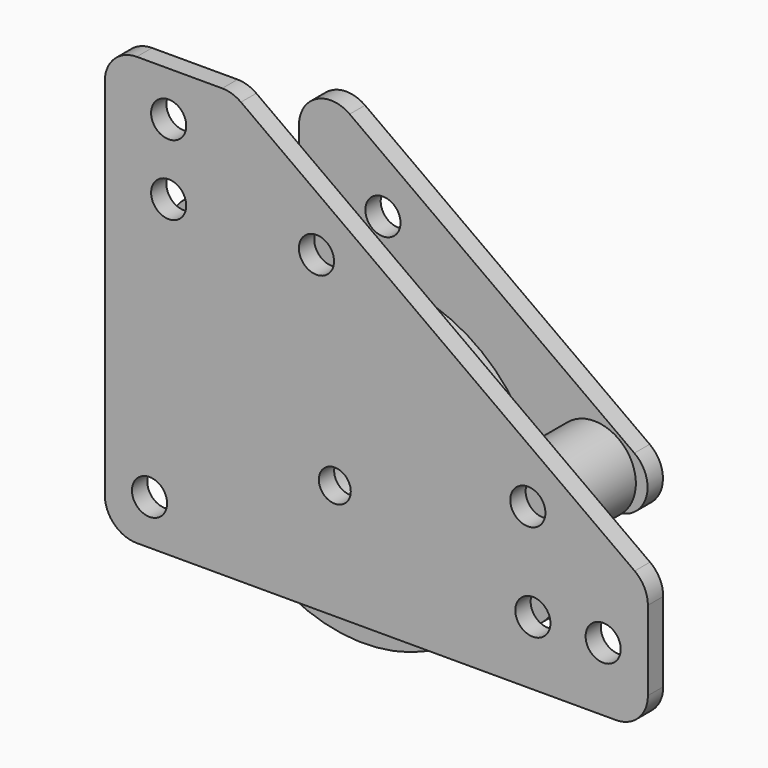
from build123d import *

# Parameters (mm, degrees)
F0_R      = 20
F0_R_2    = 13
F1_DEPTH  = 5
F0_R_3    = 24
F2_DEPTH  = 2.4
F4_R      = 2.75
F4_R_2    = 2.5
F5_DEPTH  = 3
F6_R      = 13
F6_R_2    = 5
F7_DEPTH  = 8
F8_R      = 2.75
F9_DEPTH  = 3
F10_R     = 5
F10_2_R   = 5
F11_R     = 6.5
F12_DEPTH = 10


# Not quite as in the source:
# - a feature names something its author has since deleted; it is built from what else it names


with BuildPart() as f1:
    # F0 (on Front) → F1 (new body, symmetric)
    with BuildSketch(Plane.XZ):
        Circle(F0_R)
        Circle(F0_R_2, mode=Mode.SUBTRACT)
    extrude(amount=F1_DEPTH, both=True)

    # F0 (on Front) → F2 (join, symmetric)
    with BuildSketch(Plane.XZ):
        Circle(F0_R_3)
        Circle(F0_R, mode=Mode.SUBTRACT)
    extrude(amount=F2_DEPTH, both=True)


with BuildPart() as f5:
    # F4 (on offset) → F5 (new body)
    with BuildSketch(Plane.XZ.offset(5)):
        Polygon((-16, 49), (-36, 49), (-36, -18), (49, -18), (49, 2), align=None)
        with Locations((-28.9929573972, -10.9929573972)):
            Circle(F4_R, mode=Mode.SUBTRACT)
        Circle(F4_R_2, mode=Mode.SUBTRACT)
        with Locations((31, -8)):
            Circle(F4_R, mode=Mode.SUBTRACT)
        with Locations((42, -8)):
            Circle(F4_R, mode=Mode.SUBTRACT)
        with Locations((30.2115080133, 6.9472860574)):
            Circle(F4_R, mode=Mode.SUBTRACT)
        with Locations((-26, 31)):
            Circle(F4_R, mode=Mode.SUBTRACT)
        with Locations((-2.8688968517, 30.8669634213)):
            Circle(F4_R, mode=Mode.SUBTRACT)
        with Locations((-26, 42)):
            Circle(F4_R, mode=Mode.SUBTRACT)
    extrude(amount=F5_DEPTH)

    # F10#2
    f10_2_edges = [f5.edges().sort_by_distance(p)[0] for p in [
        (-36, -6.5, 49),
        (-36, -6.5, -18),
        (49, -6.5, -18),
        (49, -6.5, 2),
        (-16, -6.5, 49),
    ]]
    fillet(f10_2_edges, radius=F10_2_R)


with BuildPart() as f7:
    # F6 (on offset) → F7 (new body)
    with BuildSketch(Plane.XZ.offset(5)):
        Circle(F6_R)
        Circle(F6_R_2, mode=Mode.SUBTRACT)
    extrude(amount=-F7_DEPTH)


with BuildPart() as f9:
    # F8 (on face) → F9 (new body)
    with BuildSketch(Plane(origin=(0, 5, 0), x_dir=(-1, 0, 0), z_dir=(0, 1, 0))):
        Polygon((-24, 2), (-24, -18), (36, -18), (36, 24), (16, 24), (16, 49), (-49, 2), align=None)
        with Locations((-30.2115080133, 6.9472860574)):
            Circle(F8_R, mode=Mode.SUBTRACT)
        with Locations((28.9929573972, -10.9929573972)):
            Circle(F8_R, mode=Mode.SUBTRACT)
        with Locations((2.8688968517, 30.8669634213)):
            Circle(F8_R, mode=Mode.SUBTRACT)
    extrude(amount=F9_DEPTH)

    # F10
    f10_edges = [f9.edges().sort_by_distance(p)[0] for p in [
        (49, 6.5, 2),
        (-16, 6.5, 49),
        (-36, 6.5, -18),
        (-36, 6.5, 24),
        (24, 6.5, -18),
    ]]
    fillet(f10_edges, radius=F10_R)


with BuildPart() as f12:
    # F11 (on face) → F12 (new body, through all)
    with BuildSketch(Plane(origin=(0, -5, 0), x_dir=(-1, 0, 0), z_dir=(0, 1, 0))):
        with Locations((-30.2115080133, 6.9472860574)):
            Circle(F11_R)
    extrude(amount=F12_DEPTH)


solid = Compound([f1.part, f5.part, f7.part, f9.part, f12.part])
